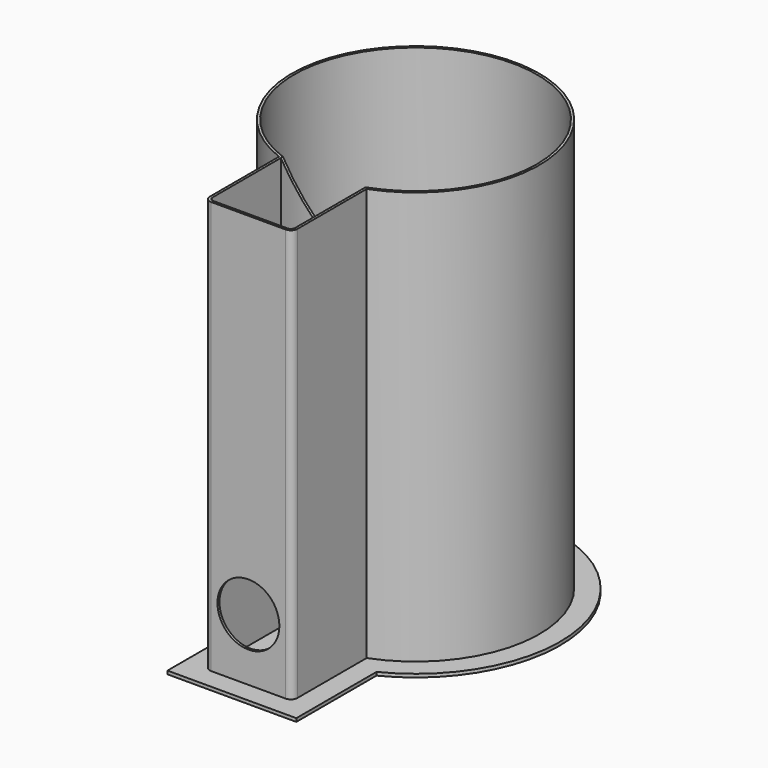
from build123d import *

# Parameters (mm, degrees)
F0_R     = 294
F1_DEPTH = 1000
F3_DEPTH = 300.001
F4_DEPTH = 1000
F2_R     = 75
F5_DEPTH = 506.001
F6_R     = 294
F7_DEPTH = 8


with BuildPart() as f1:
    # F0 (on Top) → F1 (new body)
    with BuildSketch(Plane.XY):
        with BuildLine():
            ThreePointArc((106, -280.6492472821), (246.7792535851, -170.5872210923), (300, 0))
            ThreePointArc((300, 0), (-170.5872210923, 246.7792535851), (-106, -280.6492472821))
            ThreePointArc((-106, -280.6492472821), (-103.0058387781, -281.7619512596), (-100, -282.8427124746))
            ThreePointArc((-100, -282.8427124746), (0, -300), (100, -282.8427124746))
            ThreePointArc((100, -282.8427124746), (103.0058387781, -281.7619512596), (106, -280.6492472821))
        make_face()
        Circle(F0_R, mode=Mode.SUBTRACT)
    extrude(amount=F1_DEPTH)

    # F2 (on Front) → F3 (cut, through all)
    with BuildSketch(Plane.XZ):
        Polygon((100, 1000), (-100, 1000), (0, 900), align=None)
    extrude(amount=F3_DEPTH, mode=Mode.SUBTRACT)


with BuildPart() as f4:
    # F0 (on Top) → F4 (new body)
    with BuildSketch(Plane.XY):
        with BuildLine():
            ThreePointArc((-100, -282.8427124746), (-103.0058387781, -281.7619512596), (-106, -280.6492472821))
            Line((-106, -280.6492472821), (-106, -490))
            ThreePointArc((-106, -490), (-101.313708499, -501.313708499), (-90, -506))
            Line((-90, -506), (90, -506))
            ThreePointArc((90, -506), (101.313708499, -501.313708499), (106, -490))
            Line((106, -490), (106, -280.6492472821))
            ThreePointArc((106, -280.6492472821), (103.0058387781, -281.7619512596), (100, -282.8427124746))
            Line((100, -282.8427124746), (100, -490))
            ThreePointArc((100, -490), (97.0710678119, -497.0710678119), (90, -500))
            Line((90, -500), (-90, -500))
            ThreePointArc((-90, -500), (-97.0710678119, -497.0710678119), (-100, -490))
            Line((-100, -490), (-100, -282.8427124746))
        make_face()
    extrude(amount=F4_DEPTH)

    # F2 (on Front) → F5 (cut, through all)
    with BuildSketch(Plane.XZ):
        with Locations((0, 150)):
            Circle(F2_R)
    extrude(amount=F5_DEPTH, mode=Mode.SUBTRACT)


with BuildPart() as f7:
    # F6 (on face) → F7 (new body)
    with BuildSketch(Plane.XY):
        with BuildLine():
            ThreePointArc((156, -313.3113467463), (297.5735203273, -184.2552577269), (350, 0))
            ThreePointArc((350, 0), (-184.2552577269, 297.5735203273), (-156, -313.3113467463))
            ThreePointArc((-156, -313.3113467463), (0, -350), (156, -313.3113467463))
        make_face()
        with BuildLine():
            ThreePointArc((300, 0), (246.7792535851, -170.5872210923), (106, -280.6492472821))
            ThreePointArc((106, -280.6492472821), (103.0058387781, -281.7619512596), (100, -282.8427124746))
            ThreePointArc((100, -282.8427124746), (0, -300), (-100, -282.8427124746))
            ThreePointArc((-100, -282.8427124746), (-103.0058387781, -281.7619512596), (-106, -280.6492472821))
            ThreePointArc((-106, -280.6492472821), (-170.5872210923, 246.7792535851), (300, 0))
        make_face(mode=Mode.SUBTRACT)
        with BuildLine():
            ThreePointArc((100, -282.8427124746), (103.0058387781, -281.7619512596), (106, -280.6492472821))
            ThreePointArc((106, -280.6492472821), (246.7792535851, -170.5872210923), (300, 0))
            ThreePointArc((300, 0), (-170.5872210923, 246.7792535851), (-106, -280.6492472821))
            ThreePointArc((-106, -280.6492472821), (-103.0058387781, -281.7619512596), (-100, -282.8427124746))
            ThreePointArc((-100, -282.8427124746), (0, -300), (100, -282.8427124746))
        make_face()
        Circle(F6_R, mode=Mode.SUBTRACT)
        Circle(F6_R)
        with BuildLine():
            ThreePointArc((156, -313.3113467463), (0, -350), (-156, -313.3113467463))
            Line((-156, -313.3113467463), (-156, -556))
            Line((-156, -556), (156, -556))
            Line((156, -556), (156, -313.3113467463))
        make_face()
    extrude(amount=-F7_DEPTH)


solid = Compound([f1.part, f4.part, f7.part])
